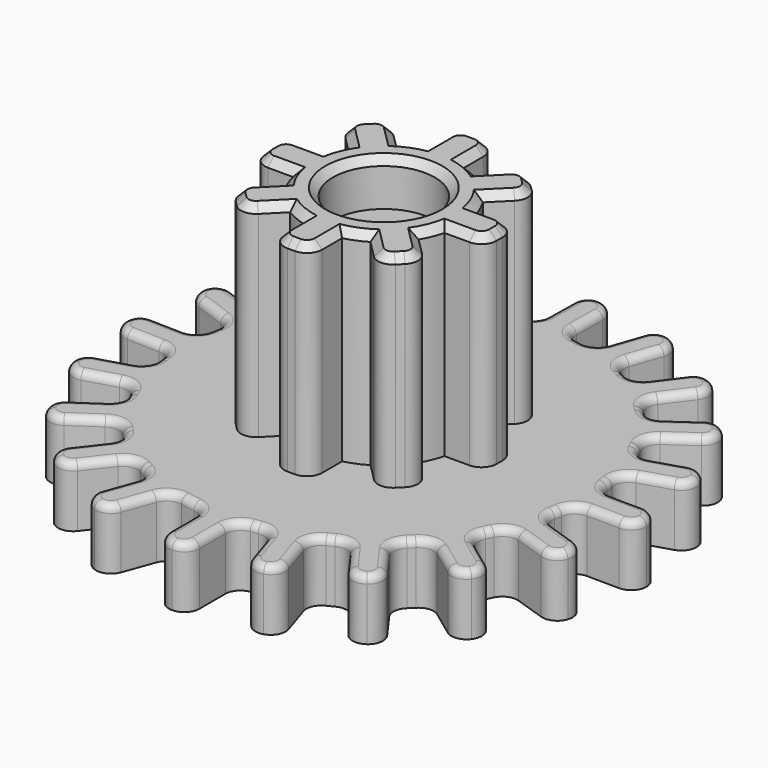
from build123d import *

# Parameters (mm, degrees)
F0_R      = 13.5
F1_DEPTH  = 4
F2_R      = 5.165
F3_DEPTH  = 17.5
F5_DEPTH  = 4
F7_DEPTH  = 14.7
F8_R      = 1
F9_R      = 1.5
F10_DEPTH = 6
F11_R     = 3.375
F12_DEPTH = 3
F13_R     = 11.5
F13_R_2   = 5
F14_DEPTH = 2.25
F15_R     = 3.5
F16_DEPTH = 10
F17_DEPTH = 2.25
F18_R     = 0.99999
F19_R     = 1
F20_SIZE  = 0.5
F21_R     = 0.5


# Not quite as in the source:
# - a fillet or chamfer is up to 0.001 mm smaller than in the source, because OpenCascade refuses the exact size


with BuildPart() as f1:
    # F0 (on Top) → F1 (new body)
    with BuildSketch(Plane.XY):
        Circle(F0_R)
    extrude(amount=F1_DEPTH)

    # F2 (on face) → F3 (join)
    with BuildSketch(Plane(origin=(0, 0, 0), x_dir=(1, 0, 0), z_dir=(0, 0, -1))):
        Circle(F2_R)
    extrude(amount=-F3_DEPTH)

    # F4 (on face) → F5 (join)
    with BuildSketch(Plane(origin=(0, 0, 0), x_dir=(1, 0, 0), z_dir=(0, 0, -1))):
        with BuildLine():
            ThreePointArc((13.4715298253, -0.8762900005), (13.4928805791, -0.4383761843), (13.5, 0))
            ThreePointArc((13.5, 0), (13.4882844657, 0.5623007836), (13.4531581968, 1.1236256185))
            Line((13.4531581968, 1.1236256185), (8.9904344714, 1.0826301377))
            Line((8.9904344714, 1.0826301377), (9.0088060999, -0.9172854813))
            Line((9.0088060999, -0.9172854813), (13.4715298253, -0.8762900005))
        make_face()
        with BuildLine():
            ThreePointArc((13.4531581968, 1.1236256185), (13.4882844657, 0.5623007836), (13.5, 0))
            ThreePointArc((13.5, 0), (13.4928805791, -0.4383761843), (13.4715298253, -0.8762900005))
            Line((13.4715298253, -0.8762900005), (17.5084474808, -0.8392060602))
            Line((17.5084474808, -0.8392060602), (17.4900758523, 1.1607095588))
            Line((17.4900758523, 1.1607095588), (13.4531581968, 1.1236256185))
        make_face()
        with BuildLine():
            Line((8.9904344714, 1.0826301377), (13.4531581968, 1.1236256185))
            ThreePointArc((13.4531581968, 1.1236256185), (13.3158775959, 2.2220269688), (13.0890696198, 3.3054888424))
            Line((13.0890696198, 3.3054888424), (8.8548373645, 1.8952190501))
            Line((8.8548373645, 1.8952190501), (8.2228420275, 3.7927389826))
            Line((8.2228420275, 3.7927389826), (12.4570742828, 5.2030087749))
            ThreePointArc((12.4570742828, 5.2030087749), (11.9889300478, 6.2060902595), (11.4401799772, 7.1674459948))
            Line((11.4401799772, 7.1674459948), (7.8441212036, 4.5243521683))
            Line((7.8441212036, 4.5243521683), (6.6596506983, 6.1358823796))
            Line((6.6596506983, 6.1358823796), (10.2557094719, 8.7789762062))
            ThreePointArc((10.2557094719, 8.7789762062), (9.5019967731, 9.5896849439), (8.6843987748, 10.3359188233))
            Line((8.6843987748, 10.3359188233), (6.0744491896, 6.7157328002))
            Line((6.0744491896, 6.7157328002), (4.4521066434, 7.885350115))
            Line((4.4521066434, 7.885350115), (7.0620562286, 11.505536138))
            ThreePointArc((7.0620562286, 11.505536138), (6.0957003372, 12.0454322213), (5.0883608871, 12.504342585))
            Line((5.0883608871, 12.504342585), (3.7170454657, 8.2573344976))
            Line((3.7170454657, 8.2573344976), (1.8138001987, 8.8718729048))
            Line((1.8138001987, 8.8718729048), (3.1851156201, 13.1188809922))
            ThreePointArc((3.1851156201, 13.1188809922), (2.0996160423, 13.3357269196), (1, 13.4629120178))
            Line((1, 13.4629120178), (1, 9))
            Line((1, 9), (-1, 9))
            Line((-1, 9), (-1, 13.4629120178))
            ThreePointArc((-1, 13.4629120178), (-2.3442503985, 13.2949046657), (-3.6648944771, 12.9930192208))
            Line((-3.6648944771, 12.9930192208), (-2.1384886691, 8.7992537304))
            Line((-2.1384886691, 8.7992537304), (-4.0178739107, 8.1152134437))
            Line((-4.0178739107, 8.1152134437), (-5.5442797187, 12.3089789341))
            ThreePointArc((-5.5442797187, 12.3089789341), (-6.5340809338, 11.8133731995), (-7.4799512018, 11.2383419604))
            Line((-7.4799512018, 11.2383419604), (-4.7387739048, 7.7164772973))
            Line((-4.7387739048, 7.7164772973), (-6.3170549236, 6.4880518719))
            Line((-6.3170549236, 6.4880518719), (-9.0582322206, 10.009916535))
            ThreePointArc((-9.0582322206, 10.009916535), (-9.8478650802, 9.2341514696), (-10.5712872446, 8.3963019236))
            Line((-10.5712872446, 8.3963019236), (-6.8805603363, 5.887095163))
            Line((-6.8805603363, 5.887095163), (-8.0050309736, 4.2331405731))
            Line((-8.0050309736, 4.2331405731), (-11.6957578819, 6.7423473336))
            ThreePointArc((-11.6957578819, 6.7423473336), (-12.2088216694, 5.7614818792), (-12.6398012119, 4.7418799355))
            Line((-12.6398012119, 4.7418799355), (-8.3566199891, 3.4881087078))
            Line((-8.3566199891, 3.4881087078), (-8.9184823887, 1.5686528881))
            Line((-8.9184823887, 1.5686528881), (-13.2016636115, 2.8224241157))
            ThreePointArc((-13.2016636115, 2.8224241157), (-13.3885169771, 1.7313616476), (-13.4853545871, 0.62865862))
            Line((-13.4853545871, 0.62865862), (-9.0241371056, 0.7516312257))
            Line((-9.0241371056, 0.7516312257), (-8.9690284209, -1.2476093883))
            Line((-8.9690284209, -1.2476093883), (-13.4302459024, -1.370581994))
            ThreePointArc((-13.4302459024, -1.370581994), (-13.2728098985, -2.4662760181), (-13.0261360789, -3.5453883924))
            Line((-13.0261360789, -3.5453883924), (-8.8185262453, -2.057570135))
            Line((-8.8185262453, -2.057570135), (-8.1517785024, -3.9431595514))
            Line((-8.1517785024, -3.9431595514), (-12.359388336, -5.4309778088))
            ThreePointArc((-12.359388336, -5.4309778088), (-11.8728956413, -6.425289806), (-11.3065772516, -7.3764022974))
            Line((-11.3065772516, -7.3764022974), (-7.7596812322, -4.6676918466))
            Line((-7.7596812322, -4.6676918466), (-6.5458054309, -6.2571903647))
            Line((-6.5458054309, -6.2571903647), (-10.0927014504, -8.9659008155))
            ThreePointArc((-10.0927014504, -8.9659008155), (-9.3242225356, -9.7626263939), (-8.4930535605, -10.4937143671))
            Line((-8.4930535605, -10.4937143671), (-5.9500503328, -6.8261922795))
            Line((-5.9500503328, -6.8261922795), (-4.3064947024, -7.9658083945))
            Line((-4.3064947024, -7.9658083945), (-6.8494979301, -11.6333304821))
            ThreePointArc((-6.8494979301, -11.6333304821), (-5.8733867675, -12.155382671), (-4.8577867393, -12.5957099044))
            Line((-4.8577867393, -12.5957099044), (-3.5647239018, -8.3242263006))
            Line((-3.5647239018, -8.3242263006), (-1.6505102284, -8.9036967595))
            Line((-1.6505102284, -8.9036967595), (-2.943573066, -13.1751803633))
            ThreePointArc((-2.943573066, -13.1751803633), (-1.8542730305, -13.3720481426), (-0.7525060589, -13.4790108922))
            Line((-0.7525060589, -13.4790108922), (-0.8344935612, -9.0168520281))
            Line((-0.8344935612, -9.0168520281), (1.1651689221, -8.9801103213))
            Line((1.1651689221, -8.9801103213), (1.2471564244, -13.4422691854))
            ThreePointArc((1.2471564244, -13.4422691854), (2.3442503985, -13.2949046657), (3.4255831444, -13.0581537792))
            Line((3.4255831444, -13.0581537792), (1.9764779811, -8.8370546445))
            Line((1.9764779811, -8.8370546445), (3.8681124645, -8.1876557061))
            Line((3.8681124645, -8.1876557061), (5.3172176278, -12.4087548408))
            ThreePointArc((5.3172176278, -12.4087548408), (6.315956506, -11.9314162367), (7.272230965, -11.373858483))
            Line((7.272230965, -11.373858483), (4.596215924, -7.8022303978))
            Line((4.596215924, -7.8022303978), (6.1967978181, -6.6030066486))
            Line((6.1967978181, -6.6030066486), (8.8728128591, -10.1746347339))
            ThreePointArc((8.8728128591, -10.1746347339), (9.6765639278, -9.4135068148), (10.4152560198, -8.5890885454))
            Line((10.4152560198, -8.5890885454), (6.7712482221, -6.0125034316))
            Line((6.7712482221, -6.0125034316), (7.9259136529, -4.3794854455))
            Line((7.9259136529, -4.3794854455), (11.5699214506, -6.9560705593))
            ThreePointArc((11.5699214506, -6.9560705593), (12.1009179897, -5.9847960538), (12.5505557587, -4.9732836384))
            Line((12.5505557587, -4.9732836384), (8.2911302059, -3.6410383009))
            Line((8.2911302059, -3.6410383009), (8.8881598279, -1.7322282971))
            Line((8.8881598279, -1.7322282971), (13.1475853807, -3.0644736347))
            ThreePointArc((13.1475853807, -3.0644736347), (13.3544509618, -1.9770279482), (13.4715298253, -0.8762900005))
            Line((13.4715298253, -0.8762900005), (9.0088060999, -0.9172854813))
            Line((9.0088060999, -0.9172854813), (8.9904344714, 1.0826301377))
        make_face()
        with BuildLine():
            Line((8.8548373645, 1.8952190501), (13.0890696198, 3.3054888424))
            ThreePointArc((13.0890696198, 3.3054888424), (12.808259544, 4.2659685246), (12.4570742828, 5.2030087749))
            Line((12.4570742828, 5.2030087749), (8.2228420275, 3.7927389826))
            Line((8.2228420275, 3.7927389826), (8.8548373645, 1.8952190501))
        make_face()
        with BuildLine():
            ThreePointArc((12.4570742828, 5.2030087749), (12.808259544, 4.2659685246), (13.0890696198, 3.3054888424))
            Line((13.0890696198, 3.3054888424), (16.9192970774, 4.5811992323))
            Line((16.9192970774, 4.5811992323), (16.2873017405, 6.4787191647))
            Line((16.2873017405, 6.4787191647), (12.4570742828, 5.2030087749))
        make_face()
        with BuildLine():
            Line((17.0006023439, -4.2696041907), (13.1475853807, -3.0644736347))
            ThreePointArc((13.1475853807, -3.0644736347), (12.8844675254, -4.0299499485), (12.5505557587, -4.9732836384))
            Line((12.5505557587, -4.9732836384), (16.4035727219, -6.1784141944))
            Line((16.4035727219, -6.1784141944), (17.0006023439, -4.2696041907))
        make_face()
        with BuildLine():
            ThreePointArc((12.5505557587, -4.9732836384), (12.8844675254, -4.0299499485), (13.1475853807, -3.0644736347))
            Line((13.1475853807, -3.0644736347), (8.8881598279, -1.7322282971))
            Line((8.8881598279, -1.7322282971), (8.2911302059, -3.6410383009))
            Line((8.2911302059, -3.6410383009), (12.5505557587, -4.9732836384))
        make_face()
        with BuildLine():
            Line((7.8441212036, 4.5243521683), (11.4401799772, 7.1674459948))
            ThreePointArc((11.4401799772, 7.1674459948), (10.8778289264, 7.995175911), (10.2557094719, 8.7789762062))
            Line((10.2557094719, 8.7789762062), (6.6596506983, 6.1358823796))
            Line((6.6596506983, 6.1358823796), (7.8441212036, 4.5243521683))
        make_face()
        with BuildLine():
            ThreePointArc((10.2557094719, 8.7789762062), (10.8778289264, 7.995175911), (11.4401799772, 7.1674459948))
            Line((11.4401799772, 7.1674459948), (14.6931246017, 9.558351816))
            Line((14.6931246017, 9.558351816), (13.5086540964, 11.1698820273))
            Line((13.5086540964, 11.1698820273), (10.2557094719, 8.7789762062))
        make_face()
        with BuildLine():
            Line((14.8662400938, -9.2868135264), (11.5699214506, -6.9560705593))
            ThreePointArc((11.5699214506, -6.9560705593), (11.0228714062, -7.7939916578), (10.4152560198, -8.5890885454))
            Line((10.4152560198, -8.5890885454), (13.711574663, -10.9198315125))
            Line((13.711574663, -10.9198315125), (14.8662400938, -9.2868135264))
        make_face()
        with BuildLine():
            ThreePointArc((10.4152560198, -8.5890885454), (11.0228714062, -7.7939916578), (11.5699214506, -6.9560705593))
            Line((11.5699214506, -6.9560705593), (7.9259136529, -4.3794854455))
            Line((7.9259136529, -4.3794854455), (6.7712482221, -6.0125034316))
            Line((6.7712482221, -6.0125034316), (10.4152560198, -8.5890885454))
        make_face()
        with BuildLine():
            Line((6.0744491896, 6.7157328002), (8.6843987748, 10.3359188233))
            ThreePointArc((8.6843987748, 10.3359188233), (7.8949168748, 10.9508121864), (7.0620562286, 11.505536138))
            Line((7.0620562286, 11.505536138), (4.4521066434, 7.885350115))
            Line((4.4521066434, 7.885350115), (6.0744491896, 6.7157328002))
        make_face()
        with BuildLine():
            ThreePointArc((7.0620562286, 11.505536138), (7.8949168748, 10.9508121864), (8.6843987748, 10.3359188233))
            Line((8.6843987748, 10.3359188233), (11.0453227774, 13.6106886212))
            Line((11.0453227774, 13.6106886212), (9.4229802312, 14.780305936))
            Line((9.4229802312, 14.780305936), (7.0620562286, 11.505536138))
        make_face()
        with BuildLine():
            Line((11.2934987518, -13.4054796983), (8.8728128591, -10.1746347339))
            ThreePointArc((8.8728128591, -10.1746347339), (8.0947603066, -10.8039277848), (7.272230965, -11.373858483))
            Line((7.272230965, -11.373858483), (9.6929168578, -14.6047034475))
            Line((9.6929168578, -14.6047034475), (11.2934987518, -13.4054796983))
        make_face()
        with BuildLine():
            ThreePointArc((7.272230965, -11.373858483), (8.0947603066, -10.8039277848), (8.8728128591, -10.1746347339))
            Line((8.8728128591, -10.1746347339), (6.1967978181, -6.6030066486))
            Line((6.1967978181, -6.6030066486), (4.596215924, -7.8022303978))
            Line((4.596215924, -7.8022303978), (7.272230965, -11.373858483))
        make_face()
        with BuildLine():
            Line((3.7170454657, 8.2573344976), (5.0883608871, 12.504342585))
            ThreePointArc((5.0883608871, 12.504342585), (4.1481342483, 12.8469055518), (3.1851156201, 13.1188809922))
            Line((3.1851156201, 13.1188809922), (1.8138001987, 8.8718729048))
            Line((1.8138001987, 8.8718729048), (3.7170454657, 8.2573344976))
        make_face()
        with BuildLine():
            ThreePointArc((3.1851156201, 13.1188809922), (4.1481342483, 12.8469055518), (5.0883608871, 12.504342585))
            Line((5.0883608871, 12.504342585), (6.3288336961, 16.3461268821))
            Line((6.3288336961, 16.3461268821), (4.4255884292, 16.9606652893))
            Line((4.4255884292, 16.9606652893), (3.1851156201, 13.1188809922))
        make_face()
        with BuildLine():
            Line((6.6280579528, -16.2271022606), (5.3172176278, -12.4087548408))
            ThreePointArc((5.3172176278, -12.4087548408), (4.3834428343, -12.768532763), (3.4255831444, -13.0581537792))
            Line((3.4255831444, -13.0581537792), (4.7364234694, -16.876501199))
            Line((4.7364234694, -16.876501199), (6.6280579528, -16.2271022606))
        make_face()
        with BuildLine():
            ThreePointArc((3.4255831444, -13.0581537792), (4.3834428343, -12.768532763), (5.3172176278, -12.4087548408))
            Line((5.3172176278, -12.4087548408), (3.8681124645, -8.1876557061))
            Line((3.8681124645, -8.1876557061), (1.9764779811, -8.8370546445))
            Line((1.9764779811, -8.8370546445), (3.4255831444, -13.0581537792))
        make_face()
        with BuildLine():
            Line((1, 9), (1, 13.4629120178))
            ThreePointArc((1, 13.4629120178), (0, 13.5), (-1, 13.4629120178))
            Line((-1, 13.4629120178), (-1, 9))
            Line((-1, 9), (1, 9))
        make_face()
        with BuildLine():
            ThreePointArc((-1, 13.4629120178), (0, 13.5), (1, 13.4629120178))
            Line((1, 13.4629120178), (1, 17.5))
            Line((1, 17.5), (-1, 17.5))
            Line((-1, 17.5), (-1, 13.4629120178))
        make_face()
        with BuildLine():
            Line((1.3213211758, -17.4786758752), (1.2471564244, -13.4422691854))
            ThreePointArc((1.2471564244, -13.4422691854), (0.2480065207, -13.497721762), (-0.7525060589, -13.4790108922))
            Line((-0.7525060589, -13.4790108922), (-0.6783413075, -17.515417582))
            Line((-0.6783413075, -17.515417582), (1.3213211758, -17.4786758752))
        make_face()
        with BuildLine():
            ThreePointArc((-0.7525060589, -13.4790108922), (0.2480065207, -13.497721762), (1.2471564244, -13.4422691854))
            Line((1.2471564244, -13.4422691854), (1.1651689221, -8.9801103213))
            Line((1.1651689221, -8.9801103213), (-0.8344935612, -9.0168520281))
            Line((-0.8344935612, -9.0168520281), (-0.7525060589, -13.4790108922))
        make_face()
        with BuildLine():
            Line((-2.1384886691, 8.7992537304), (-3.6648944771, 12.9930192208))
            ThreePointArc((-3.6648944771, 12.9930192208), (-4.6172719349, 12.6858503806), (-5.5442797187, 12.3089789341))
            Line((-5.5442797187, 12.3089789341), (-4.0178739107, 8.1152134437))
            Line((-4.0178739107, 8.1152134437), (-2.1384886691, 8.7992537304))
        make_face()
        with BuildLine():
            ThreePointArc((-5.5442797187, 12.3089789341), (-4.6172719349, 12.6858503806), (-3.6648944771, 12.9930192208))
            Line((-3.6648944771, 12.9930192208), (-5.0456598874, 16.7866410071))
            Line((-5.0456598874, 16.7866410071), (-6.925045129, 16.1026007204))
            Line((-6.925045129, 16.1026007204), (-5.5442797187, 12.3089789341))
        make_face()
        with BuildLine():
            Line((-4.1132596788, -17.0391048713), (-2.943573066, -13.1751803633))
            ThreePointArc((-2.943573066, -13.1751803633), (-3.9114255977, -12.9209422951), (-4.8577867393, -12.5957099044))
            Line((-4.8577867393, -12.5957099044), (-6.0274733522, -16.4596344124))
            Line((-6.0274733522, -16.4596344124), (-4.1132596788, -17.0391048713))
        make_face()
        with BuildLine():
            ThreePointArc((-4.8577867393, -12.5957099044), (-3.9114255977, -12.9209422951), (-2.943573066, -13.1751803633))
            Line((-2.943573066, -13.1751803633), (-1.6505102284, -8.9036967595))
            Line((-1.6505102284, -8.9036967595), (-3.5647239018, -8.3242263006))
            Line((-3.5647239018, -8.3242263006), (-4.8577867393, -12.5957099044))
        make_face()
        with BuildLine():
            Line((-4.7387739048, 7.7164772973), (-7.4799512018, 11.2383419604))
            ThreePointArc((-7.4799512018, 11.2383419604), (-8.2918716213, 10.6533968769), (-9.0582322206, 10.009916535))
            Line((-9.0582322206, 10.009916535), (-6.3170549236, 6.4880518719))
            Line((-6.3170549236, 6.4880518719), (-4.7387739048, 7.7164772973))
        make_face()
        with BuildLine():
            ThreePointArc((-9.0582322206, 10.009916535), (-8.2918716213, 10.6533968769), (-7.4799512018, 11.2383419604))
            Line((-7.4799512018, 11.2383419604), (-9.9595819627, 14.4241716271))
            Line((-9.9595819627, 14.4241716271), (-11.5378629815, 13.1957462017))
            Line((-11.5378629815, 13.1957462017), (-9.0582322206, 10.009916535))
        make_face()
        with BuildLine():
            Line((-9.1498631912, -14.950919824), (-6.8494979301, -11.6333304821))
            ThreePointArc((-6.8494979301, -11.6333304821), (-7.6924087764, -11.0940005055), (-8.4930535605, -10.4937143671))
            Line((-8.4930535605, -10.4937143671), (-10.7934188217, -13.8113037089))
            Line((-10.7934188217, -13.8113037089), (-9.1498631912, -14.950919824))
        make_face()
        with BuildLine():
            ThreePointArc((-8.4930535605, -10.4937143671), (-7.6924087764, -11.0940005055), (-6.8494979301, -11.6333304821))
            Line((-6.8494979301, -11.6333304821), (-4.3064947024, -7.9658083945))
            Line((-4.3064947024, -7.9658083945), (-5.9500503328, -6.8261922795))
            Line((-5.9500503328, -6.8261922795), (-8.4930535605, -10.4937143671))
        make_face()
        with BuildLine():
            Line((-6.8805603363, 5.887095163), (-10.5712872446, 8.3963019236))
            ThreePointArc((-10.5712872446, 8.3963019236), (-11.1641934824, 7.5901768021), (-11.6957578819, 6.7423473336))
            Line((-11.6957578819, 6.7423473336), (-8.0050309736, 4.2331405731))
            Line((-8.0050309736, 4.2331405731), (-6.8805603363, 5.887095163))
        make_face()
        with BuildLine():
            ThreePointArc((-11.6957578819, 6.7423473336), (-11.1641934824, 7.5901768021), (-10.5712872446, 8.3963019236))
            Line((-10.5712872446, 8.3963019236), (-13.9098673437, 10.6660953718))
            Line((-13.9098673437, 10.6660953718), (-15.0343379811, 9.0121407818))
            Line((-15.0343379811, 9.0121407818), (-11.6957578819, 6.7423473336))
        make_face()
        with BuildLine():
            Line((-13.301174133, -11.41616252), (-10.0927014504, -8.9659008155))
            ThreePointArc((-10.0927014504, -8.9659008155), (-10.7291149974, -8.1936616585), (-11.3065772516, -7.3764022974))
            Line((-11.3065772516, -7.3764022974), (-14.5150499342, -9.8266640019))
            Line((-14.5150499342, -9.8266640019), (-13.301174133, -11.41616252))
        make_face()
        with BuildLine():
            ThreePointArc((-11.3065772516, -7.3764022974), (-10.7291149974, -8.1936616585), (-10.0927014504, -8.9659008155))
            Line((-10.0927014504, -8.9659008155), (-6.5458054309, -6.2571903647))
            Line((-6.5458054309, -6.2571903647), (-7.7596812322, -4.6676918466))
            Line((-7.7596812322, -4.6676918466), (-11.3065772516, -7.3764022974))
        make_face()
        with BuildLine():
            Line((-8.3566199891, 3.4881087078), (-12.6398012119, 4.7418799355))
            ThreePointArc((-12.6398012119, 4.7418799355), (-12.9563267833, 3.7925711969), (-13.2016636115, 2.8224241157))
            Line((-13.2016636115, 2.8224241157), (-8.9184823887, 1.5686528881))
            Line((-8.9184823887, 1.5686528881), (-8.3566199891, 3.4881087078))
        make_face()
        with BuildLine():
            ThreePointArc((-13.2016636115, 2.8224241157), (-12.9563267833, 3.7925711969), (-12.6398012119, 4.7418799355))
            Line((-12.6398012119, 4.7418799355), (-16.514307223, 5.8760239059))
            Line((-16.514307223, 5.8760239059), (-17.0761696226, 3.9565680862))
            Line((-17.0761696226, 3.9565680862), (-13.2016636115, 2.8224241157))
        make_face()
        with BuildLine():
            Line((-16.1655335221, -6.7768374589), (-12.359388336, -5.4309778088))
            ThreePointArc((-12.359388336, -5.4309778088), (-12.7277285608, -4.5005472648), (-13.0261360789, -3.5453883924))
            Line((-13.0261360789, -3.5453883924), (-16.8322812651, -4.8912480425))
            Line((-16.8322812651, -4.8912480425), (-16.1655335221, -6.7768374589))
        make_face()
        with BuildLine():
            ThreePointArc((-13.0261360789, -3.5453883924), (-12.7277285608, -4.5005472648), (-12.359388336, -5.4309778088))
            Line((-12.359388336, -5.4309778088), (-8.1517785024, -3.9431595514))
            Line((-8.1517785024, -3.9431595514), (-8.8185262453, -2.057570135))
            Line((-8.8185262453, -2.057570135), (-13.0261360789, -3.5453883924))
        make_face()
        with BuildLine():
            Line((-9.0241371056, 0.7516312257), (-13.4853545871, 0.62865862))
            ThreePointArc((-13.4853545871, 0.62865862), (-13.4948741448, -0.371983622), (-13.4302459024, -1.370581994))
            Line((-13.4302459024, -1.370581994), (-8.9690284209, -1.2476093883))
            Line((-8.9690284209, -1.2476093883), (-9.0241371056, 0.7516312257))
        make_face()
        with BuildLine():
            ThreePointArc((-13.4302459024, -1.370581994), (-13.4948741448, -0.371983622), (-13.4853545871, 0.62865862))
            Line((-13.4853545871, 0.62865862), (-17.5209097153, 0.5174193156))
            Line((-17.5209097153, 0.5174193156), (-17.4658010306, -1.4818212985))
            Line((-17.4658010306, -1.4818212985), (-13.4302459024, -1.370581994))
        make_face()
    extrude(amount=-F5_DEPTH)

    # F6 (on face) → F7 (join)
    with BuildSketch(Plane.XY.offset(17.5)):
        Polygon((3.017766953, -1.25), (7.665, -1.25), (7.665, 1.25), (3.017766953, 1.25), (2.7683230483, 1.0005560954), (2.665, 1.1038791437), (2.665, -1.1038791437), (2.7683230483, -1.0005560954), align=None)
        Polygon((6.3038569543, -4.5360900013), (3.017766953, -1.25), (2.665, -1.25), (2.665, -1.1038791437), (1.1038791437, -2.665), (1.25, -2.665), (1.25, -3.017766953), (4.5360900013, -6.3038569543), align=None)
        Polygon((2.665, -1.25), (3.017766953, -1.25), (2.7683230483, -1.0005560954), (2.665, -1.1038791437), align=None)
        Polygon((2.7683230483, 1.0005560954), (3.017766953, 1.25), (2.665, 1.25), (2.665, 1.1038791437), align=None)
        Polygon((2.665, 1.25), (3.017766953, 1.25), (6.3038569543, 4.5360900013), (4.5360900013, 6.3038569543), (1.25, 3.017766953), (1.25, 2.665), (1.1038791437, 2.665), (2.665, 1.1038791437), align=None)
        Polygon((1.0005560954, -2.7683230483), (1.1038791437, -2.665), (-1.1038791437, -2.665), (-1.0005560954, -2.7683230483), (-1.25, -3.017766953), (-1.25, -7.665), (1.25, -7.665), (1.25, -3.017766953), align=None)
        Polygon((1.25, -2.665), (1.1038791437, -2.665), (1.0005560954, -2.7683230483), (1.25, -3.017766953), align=None)
        Polygon((-1.1038791437, 2.665), (1.1038791437, 2.665), (1.0005560954, 2.7683230483), (1.25, 3.017766953), (1.25, 7.665), (-1.25, 7.665), (-1.25, 3.017766953), (-1.0005560954, 2.7683230483), align=None)
        Polygon((1.0005560954, 2.7683230483), (1.1038791437, 2.665), (1.25, 2.665), (1.25, 3.017766953), align=None)
        Polygon((-1.25, -2.665), (-1.1038791437, -2.665), (-2.665, -1.1038791437), (-2.665, -1.25), (-3.017766953, -1.25), (-6.3038569543, -4.5360900013), (-4.5360900013, -6.3038569543), (-1.25, -3.017766953), align=None)
        Polygon((-1.0005560954, -2.7683230483), (-1.1038791437, -2.665), (-1.25, -2.665), (-1.25, -3.017766953), align=None)
        Polygon((-2.665, 1.1038791437), (-1.1038791437, 2.665), (-1.25, 2.665), (-1.25, 3.017766953), (-4.5360900013, 6.3038569543), (-6.3038569543, 4.5360900013), (-3.017766953, 1.25), (-2.665, 1.25), align=None)
        Polygon((-1.25, 2.665), (-1.1038791437, 2.665), (-1.0005560954, 2.7683230483), (-1.25, 3.017766953), align=None)
        Polygon((-2.7683230483, -1.0005560954), (-2.665, -1.1038791437), (-2.665, 1.1038791437), (-2.7683230483, 1.0005560954), (-3.017766953, 1.25), (-7.665, 1.25), (-7.665, -1.25), (-3.017766953, -1.25), align=None)
        Polygon((-2.665, -1.25), (-2.665, -1.1038791437), (-2.7683230483, -1.0005560954), (-3.017766953, -1.25), align=None)
        Polygon((-2.7683230483, 1.0005560954), (-2.665, 1.1038791437), (-2.665, 1.25), (-3.017766953, 1.25), align=None)
    extrude(amount=-F7_DEPTH)

    # F8
    f8_edges = [f1.edges().sort_by_distance(p)[0] for p in [
        (1.25, -7.665, 10.75),
        (-1.25, -7.665, 10.75),
        (-4.53609, -6.303857, 10.75),
        (-6.303857, -4.53609, 10.75),
        (-7.665, -1.25, 10.75),
        (-7.665, 1.25, 10.75),
        (-6.303857, 4.53609, 10.75),
        (-4.53609, 6.303857, 10.75),
        (-1.25, 7.665, 10.75),
        (1.25, 7.665, 10.75),
        (4.53609, 6.303857, 10.75),
        (6.303857, 4.53609, 10.75),
        (7.665, 1.25, 10.75),
        (7.665, -1.25, 10.75),
        (6.303857, -4.53609, 10.75),
        (4.53609, -6.303857, 10.75),
    ]]
    fillet(f8_edges, radius=F8_R)

    # F9 (on face) → F10 (cut)
    with BuildSketch(Plane.XY.offset(17.5)):
        Circle(F9_R)
    extrude(amount=-F10_DEPTH, mode=Mode.SUBTRACT)

    # F11 (on face) → F12 (cut)
    with BuildSketch(Plane.XY.offset(17.5)):
        Circle(F11_R)
    extrude(amount=-F12_DEPTH, mode=Mode.SUBTRACT)

    # F13 (on face) → F14 (cut)
    with BuildSketch(Plane(origin=(0, 0, 0), x_dir=(1, 0, 0), z_dir=(0, 0, -1))):
        Circle(F13_R)
        Circle(F13_R_2, mode=Mode.SUBTRACT)
    extrude(amount=-F14_DEPTH, mode=Mode.SUBTRACT)

    # F15 (on face) → F16 (cut)
    with BuildSketch(Plane(origin=(0, 0, 0), x_dir=(1, 0, 0), z_dir=(0, 0, -1))):
        Circle(F15_R)
    extrude(amount=-F16_DEPTH, mode=Mode.SUBTRACT)

    # F17 (add): a face of the model
    f17_faces = [f1.faces().sort_by_distance(p)[0] for p in [
        (-11.1747308807, 0, 2.25),
    ]]
    extrude(f17_faces, amount=F17_DEPTH)

    # F18 (radius 1 in the source; OpenCascade refuses exactly that, so slightly less here)
    f18_edges = [f1.edges().sort_by_distance(p)[0] for p in [
        (14.693125, -9.558352, 2),
        (13.508654, -11.169882, 2),
        (16.287302, -6.478719, 2),
        (16.919297, -4.581199, 2),
        (17.490076, -1.16071, 2),
        (17.508447, 0.839206, 2),
        (17.000602, 4.269604, 2),
        (16.403573, 6.178414, 2),
        (14.86624, 9.286814, 2),
        (13.711575, 10.919832, 2),
        (11.293499, 13.40548, 2),
        (9.692917, 14.604703, 2),
        (6.628058, 16.227102, 2),
        (4.736423, 16.876501, 2),
        (1.321321, 17.478676, 2),
        (-0.678341, 17.515418, 2),
        (-4.11326, 17.039105, 2),
        (-6.027473, 16.459634, 2),
        (-9.149863, 14.95092, 2),
        (-10.793419, 13.811304, 2),
        (-13.301174, 11.416163, 2),
        (-14.51505, 9.826664, 2),
        (-16.165534, 6.776837, 2),
        (-16.832281, 4.891248, 2),
        (-17.465801, 1.481821, 2),
        (-17.52091, -0.517419, 2),
        (-17.07617, -3.956568, 2),
        (-16.514307, -5.876024, 2),
        (-15.034338, -9.012141, 2),
        (-13.909867, -10.666095, 2),
        (-11.537863, -13.195746, 2),
        (-9.959582, -14.424172, 2),
        (-6.925045, -16.102601, 2),
        (-5.04566, -16.786641, 2),
        (-1, -17.5, 2),
        (1, -17.5, 2),
        (4.425588, -16.960665, 2),
        (6.328834, -16.346127, 2),
        (11.045323, -13.610689, 2),
        (9.42298, -14.780306, 2),
    ]]
    fillet(f18_edges, radius=F18_R)

    # F19
    f19_edges = [f1.edges().sort_by_distance(p)[0] for p in [
        (10.415256, 8.589089, 2),
        (8.872813, 10.174635, 2),
        (7.272231, 11.373858, 2),
        (5.317218, 12.408755, 2),
        (3.425583, 13.058154, 2),
        (1.247156, 13.442269, 2),
        (-6.849498, 11.63333, 2),
        (-0.752506, 13.479011, 2),
        (-4.857787, 12.59571, 2),
        (-2.943573, 13.17518, 2),
        (-10.092701, 8.965901, 2),
        (-8.493054, 10.493714, 2),
        (-11.306577, 7.376402, 2),
        (-12.359388, 5.430978, 2),
        (-13.026136, 3.545388, 2),
        (-13.430246, 1.370582, 2),
        (-13.485355, -0.628659, 2),
        (-12.639801, -4.74188, 2),
        (-13.201664, -2.822424, 2),
        (-11.695758, -6.742347, 2),
        (-10.571287, -8.396302, 2),
        (-9.058232, -10.009917, 2),
        (-7.479951, -11.238342, 2),
        (-3.664894, -12.993019, 2),
        (-1, -13.462912, 2),
        (1, -13.462912, 2),
        (5.088361, -12.504343, 2),
        (7.062056, -11.505536, 2),
        (3.185116, -13.118881, 2),
        (8.684399, -10.335919, 2),
        (10.255709, -8.778976, 2),
        (11.44018, -7.167446, 2),
        (12.457074, -5.203009, 2),
        (13.08907, -3.305489, 2),
        (11.569921, 6.956071, 2),
        (13.147585, 3.064474, 2),
        (13.47153, 0.87629, 2),
        (13.453158, -1.123626, 2),
        (12.550556, 4.973284, 2),
        (-5.54428, -12.308979, 2),
    ]]
    fillet(f19_edges, radius=F19_R)

    # F20
    f20_edges = [f1.edges().sort_by_distance(p)[0] for p in [
        (5.83823, 1.25, 17.5),
        (7.372107, 0.957107, 17.5),
        (4.771838, 1.97656, 17.5),
        (7.665, 0, 17.5),
        (5.012135, 3.244368, 17.5),
        (7.372107, -0.957107, 17.5),
        (5.889643, 4.53609, 17.5),
        (5.83823, -1.25, 17.5),
        (5.419973, 5.419973, 17.5),
        (4.771838, -1.97656, 17.5),
        (4.53609, 5.889643, 17.5),
        (5.012135, -3.244368, 17.5),
        (3.244368, 5.012135, 17.5),
        (5.889643, -4.53609, 17.5),
        (1.97656, 4.771838, 17.5),
        (5.419973, -5.419973, 17.5),
        (1.25, 5.83823, 17.5),
        (4.53609, -5.889643, 17.5),
        (0.957107, 7.372107, 17.5),
        (3.244368, -5.012135, 17.5),
        (0, 7.665, 17.5),
        (1.97656, -4.771838, 17.5),
        (-0.957107, 7.372107, 17.5),
        (1.25, -5.83823, 17.5),
        (-1.25, 5.83823, 17.5),
        (0.957107, -7.372107, 17.5),
        (-1.97656, 4.771838, 17.5),
        (0, -7.665, 17.5),
        (-3.244368, 5.012135, 17.5),
        (-0.957107, -7.372107, 17.5),
        (-4.53609, 5.889643, 17.5),
        (-1.25, -5.83823, 17.5),
        (-5.419973, 5.419973, 17.5),
        (-1.97656, -4.771838, 17.5),
        (-5.889643, 4.53609, 17.5),
        (-3.244368, -5.012135, 17.5),
        (-5.012135, 3.244368, 17.5),
        (-4.53609, -5.889643, 17.5),
        (-4.771838, 1.97656, 17.5),
        (-5.419973, -5.419973, 17.5),
        (-5.83823, 1.25, 17.5),
        (-5.889643, -4.53609, 17.5),
        (-7.372107, 0.957107, 17.5),
        (-5.012135, -3.244368, 17.5),
        (-7.665, 0, 17.5),
        (-4.771838, -1.97656, 17.5),
        (-7.372107, -0.957107, 17.5),
        (-5.83823, -1.25, 17.5),
        (-3.375, 0, 17.5),
    ]]
    chamfer(f20_edges, length=F20_SIZE)

    # F21
    f21_edges = [f1.edges().sort_by_distance(p)[0] for p in [
        (9.835183, -11.932139, 4),
    ]]
    fillet(f21_edges, radius=F21_R)


solid = f1.part
